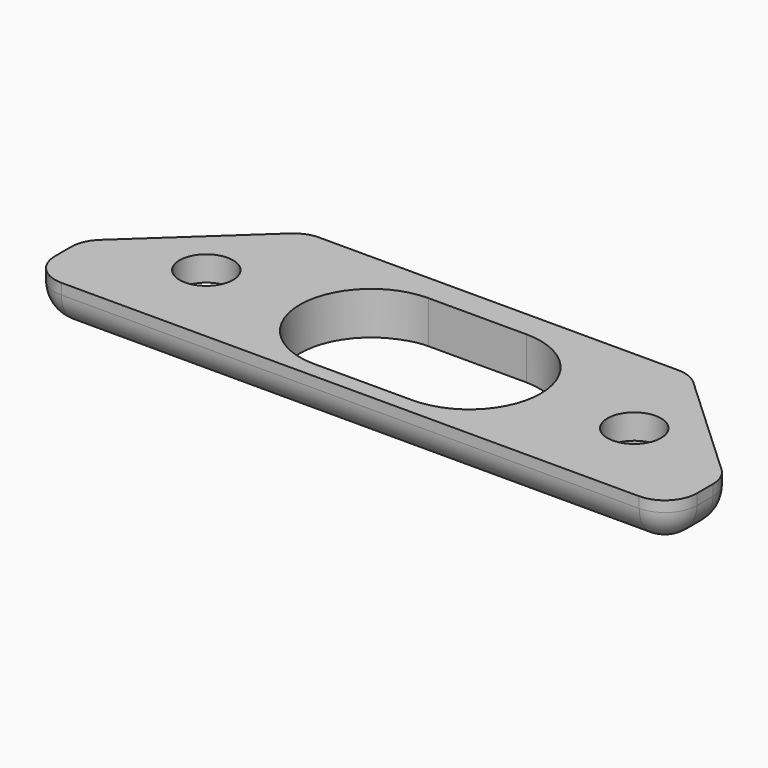
from build123d import *

# Parameters (mm, degrees)
F0_R         = 3
F0_R_2       = 1.5
F1_DEPTH     = 2.4
F2_DEPTH     = 1
F3_T1_DEPTH  = 1.1190522621
F3_T3_DEPTH  = 32.4
F3_T5_DEPTH  = 20.138628613
F3_T7_DEPTH  = 2.365520331
F3_T9_DEPTH  = 8.3614446785
F3_T11_DEPTH = 8.3614446785
F3_T13_DEPTH = 5.1
F3_T15_DEPTH = 2.5639483811
F3_T20_DEPTH = 1.8
F3_S25_W     = 1.8
F3_S25_H     = 1.8
F3_T26_DEPTH = 1.8
F3_S31_W     = 1.8
F3_S31_H     = 1.8
F3_T32_DEPTH = 1.8
F3_T38_DEPTH = 1.8
F3_T44_DEPTH = 1.8
F3_T50_DEPTH = 1.8


# Not quite as in the source:
# - a fillet or chamfer that OpenCascade refuses, or shapes differently, is made with other operations: its cross-section is extruded or revolved along the edge and cut away or added


with BuildPart() as f1:
    # F0 (on Top) → F1 (new body)
    with BuildSketch(Plane.XY):
        Polygon((-18, -1.2002319389), (-18, -4.9048635534), (18, -4.9048635534), (18, -1.2002319389), (10.7755224389, 5.5), (-10.7755224389, 5.5), align=None)
        with Locations((-12, 0)):
            Circle(F0_R, mode=Mode.SUBTRACT)
        with BuildLine():
            ThreePointArc((-2.75, -4), (-6.75, 0), (-2.75, 4))
            Line((-2.75, 4), (2.75, 4))
            ThreePointArc((2.75, 4), (6.75, 0), (2.75, -4))
            Line((2.75, -4), (-2.75, -4))
        make_face(mode=Mode.SUBTRACT)
        with Locations((12, 0)):
            Circle(F0_R, mode=Mode.SUBTRACT)
        with Locations((-12, 0)):
            Circle(F0_R)
        with Locations((-12, 0)):
            Circle(F0_R_2, mode=Mode.SUBTRACT)
        with Locations((12, 0)):
            Circle(F0_R)
        with Locations((12, 0)):
            Circle(F0_R_2, mode=Mode.SUBTRACT)
    extrude(amount=F1_DEPTH)

    # F0 (on Top) → F2 (cut)
    with BuildSketch(Plane.XY):
        with Locations((12, 0)):
            Circle(F0_R)
        with Locations((12, 0)):
            Circle(F0_R_2, mode=Mode.SUBTRACT)
        with Locations((-12, 0)):
            Circle(F0_R)
        with Locations((-12, 0)):
            Circle(F0_R_2, mode=Mode.SUBTRACT)
    extrude(amount=F2_DEPTH, mode=Mode.SUBTRACT)

    # F3: fillet of radius 1.8 on 12 edges, made by hand

    # F3_s2 → F3_t1 (cut)
    with BuildSketch(Plane.XZ.offset(1.9858112913)):
        with BuildLine():
            ThreePointArc((-18, 1.8), (-17.4727922061, 0.5272077939), (-16.2, 0))
            Line((-16.2, 0), (-18, 0))
            Line((-18, 0), (-18, 1.8))
        make_face()
        with BuildLine():
            ThreePointArc((16.2, 0), (17.4727922061, 0.5272077939), (18, 1.8))
            Line((18, 1.8), (18, 0))
            Line((18, 0), (16.2, 0))
        make_face()
    extrude(amount=F3_T1_DEPTH, mode=Mode.SUBTRACT)

    # F3_s4 → F3_t3 (cut)
    with BuildSketch(Plane.YZ.offset(-16.2)):
        with BuildLine():
            ThreePointArc((-4.9048635534, 1.8), (-4.3776557595, 0.5272077939), (-3.1048635534, 0))
            Line((-3.1048635534, 0), (-4.9048635534, 0))
            Line((-4.9048635534, 0), (-4.9048635534, 1.8))
        make_face()
    extrude(amount=F3_T3_DEPTH, mode=Mode.SUBTRACT)

    # F3_s6 → F3_t5 (cut)
    with BuildSketch(Plane.YZ.offset(-10.0693143065)):
        with BuildLine():
            ThreePointArc((3.7, 0), (4.9727922061, 0.5272077939), (5.5, 1.8))
            Line((5.5, 1.8), (5.5, 0))
            Line((5.5, 0), (3.7, 0))
        make_face()
    extrude(amount=F3_T5_DEPTH, mode=Mode.SUBTRACT)

    # F3_s8 → F3_t7 (cut)
    with BuildSketch(Plane.XY.offset(1.8)):
        with BuildLine():
            ThreePointArc((10.0693143065, 5.5), (10.7267347006, 5.3756486581), (11.2933205301, 5.0197760282))
            Line((11.2933205301, 5.0197760282), (10.7755224389, 5.5))
            Line((10.7755224389, 5.5), (10.0693143065, 5.5))
        make_face()
        with BuildLine():
            ThreePointArc((-11.2933205301, 5.0197760282), (-10.7267347006, 5.3756486581), (-10.0693143065, 5.5))
            Line((-10.0693143065, 5.5), (-10.7755224389, 5.5))
            Line((-10.7755224389, 5.5), (-11.2933205301, 5.0197760282))
        make_face()
    extrude(amount=F3_T7_DEPTH, mode=Mode.SUBTRACT)

    # F3_s10 → F3_t9 (cut)
    with BuildSketch(Plane(origin=(-3.5684530391, -3.3095075488, 0), x_dir=(0, 0, 1), z_dir=(-0.7332089046, -0.6800034575, 0))):
        with BuildLine():
            ThreePointArc((1.8, 11.3600414903), (0.5272077939, 10.8328336964), (0, 9.5600414903))
            Line((0, 9.5600414903), (0, 11.3600414903))
            Line((0, 11.3600414903), (1.8, 11.3600414903))
        make_face()
    extrude(amount=F3_T9_DEPTH, mode=Mode.SUBTRACT)

    # F3_s12 → F3_t11 (cut)
    with BuildSketch(Plane(origin=(9.6991387326, -8.9953188401, 0), x_dir=(0, 0, 1), z_dir=(-0.7332089046, 0.6800034575, 0))):
        with BuildLine():
            ThreePointArc((0, 9.5600414903), (0.5272077939, 10.8328336964), (1.8, 11.3600414903))
            Line((1.8, 11.3600414903), (0, 11.3600414903))
            Line((0, 11.3600414903), (0, 9.5600414903))
        make_face()
    extrude(amount=F3_T11_DEPTH, mode=Mode.SUBTRACT)

    # F3_s14 → F3_t13 (cut)
    with BuildSketch(Plane.XY.offset(1.8)):
        with BuildLine():
            ThreePointArc((-18, -3.1048635534), (-17.4727922061, -4.3776557595), (-16.2, -4.9048635534))
            Line((-16.2, -4.9048635534), (-18, -4.9048635534))
            Line((-18, -4.9048635534), (-18, -3.1048635534))
        make_face()
        with BuildLine():
            ThreePointArc((16.2, -4.9048635534), (17.4727922061, -4.3776557595), (18, -3.1048635534))
            Line((18, -3.1048635534), (18, -4.9048635534))
            Line((18, -4.9048635534), (16.2, -4.9048635534))
        make_face()
    extrude(amount=F3_T13_DEPTH, mode=Mode.SUBTRACT)

    # F3_s16 → F3_t15 (cut)
    with BuildSketch(Plane.XY.offset(1.8)):
        with BuildLine():
            ThreePointArc((-18, -1.9858112913), (-17.8497289478, -1.265815181), (-17.4240062235, -0.666035263))
            Line((-17.4240062235, -0.666035263), (-18, -1.2002319389))
            Line((-18, -1.2002319389), (-18, -1.9858112913))
        make_face()
        with BuildLine():
            ThreePointArc((18, -1.9858112913), (17.8497289478, -1.265815181), (17.4240062235, -0.666035263))
            Line((17.4240062235, -0.666035263), (18, -1.2002319389))
            Line((18, -1.2002319389), (18, -1.9858112913))
        make_face()
    extrude(amount=F3_T15_DEPTH, mode=Mode.SUBTRACT)


with BuildPart() as f3_tool18:
    # F3_s19 → F3_t20 (new body)
    with BuildSketch(Plane.XY.offset(1.8)):
        Polygon((-16.2, -1.9858112913), (-18, -1.9858112913), (-18, -1.2002319389), (-17.4240062235, -0.666035263), align=None)
    extrude(amount=-F3_T20_DEPTH)

    # F3_s21 → F3_t22 (revolve, cut)
    with BuildSketch(Plane(origin=(-16.2, -1.9858112913, 1.8), x_dir=(0.9165160821, -0.399997839, 0), z_dir=(0.399997839, 0.9165160821, 0))):
        with BuildLine():
            ThreePointArc((0, -1.8), (1.8, 0), (0, 1.8))
            Line((0, 1.8), (0, -1.8))
        make_face()
    revolve(axis=Axis((-16.2, -1.9858112913, 1.8), (0, 0, -1)), mode=Mode.SUBTRACT)


with BuildPart() as f1_1:
    add(f1.part)

    # F3_t17: cut F3_tool18
    add(f3_tool18.part, mode=Mode.SUBTRACT)


with BuildPart() as f3_tool24:
    # F3_s25 → F3_t26 (new body)
    with BuildSketch(Plane.YZ.offset(-16.2)):
        with Locations((-4.0048635534, 0.9)):
            Rectangle(F3_S25_W, F3_S25_H)
    extrude(amount=-F3_T26_DEPTH)

    # F3_s27 → F3_t28 (revolve, cut)
    with BuildSketch(Plane(origin=(-16.2, -3.1048635534, 1.8), x_dir=(0, 0.7071067812, 0.7071067812), z_dir=(0, -0.7071067812, 0.7071067812))):
        with BuildLine():
            ThreePointArc((0, -1.8), (1.8, 0), (0, 1.8))
            Line((0, 1.8), (0, -1.8))
        make_face()
    revolve(axis=Axis((-16.2, -3.1048635534, 1.8), (-1, 0, 0)), mode=Mode.SUBTRACT)


with BuildPart() as f1_2:
    add(f1_1.part)

    # F3_t23: cut F3_tool24
    add(f3_tool24.part, mode=Mode.SUBTRACT)


with BuildPart() as f3_tool30:
    # F3_s31 → F3_t32 (new body)
    with BuildSketch(Plane.XZ.offset(3.1048635534)):
        with Locations((17.1, 0.9)):
            Rectangle(F3_S31_W, F3_S31_H)
    extrude(amount=F3_T32_DEPTH)

    # F3_s33 → F3_t34 (revolve, cut)
    with BuildSketch(Plane(origin=(16.2, -3.1048635534, 1.8), x_dir=(-0.7071067812, 0, 0.7071067812), z_dir=(0.7071067812, 0, 0.7071067812))):
        with BuildLine():
            ThreePointArc((0, -1.8), (1.8, 0), (0, 1.8))
            Line((0, 1.8), (0, -1.8))
        make_face()
    revolve(axis=Axis((16.2, -3.1048635534, 1.8), (0, -1, 0)), mode=Mode.SUBTRACT)


with BuildPart() as f1_3:
    add(f1_2.part)

    # F3_t29: cut F3_tool30
    add(f3_tool30.part, mode=Mode.SUBTRACT)


with BuildPart() as f3_tool36:
    # F3_s37 → F3_t38 (new body)
    with BuildSketch(Plane.XY.offset(1.8)):
        Polygon((16.2, -1.9858112913), (18, -1.9858112913), (18, -1.2002319389), (17.4240062235, -0.666035263), align=None)
    extrude(amount=-F3_T38_DEPTH)

    # F3_s39 → F3_t40 (revolve, cut)
    with BuildSketch(Plane(origin=(16.2, -1.9858112913, 1.8), x_dir=(-0.9165160821, -0.399997839, 0), z_dir=(0.399997839, -0.9165160821, 0))):
        with BuildLine():
            ThreePointArc((0, -1.8), (1.8, 0), (0, 1.8))
            Line((0, 1.8), (0, -1.8))
        make_face()
    revolve(axis=Axis((16.2, -1.9858112913, 1.8), (0, 0, -1)), mode=Mode.SUBTRACT)


with BuildPart() as f1_4:
    add(f1_3.part)

    # F3_t35: cut F3_tool36
    add(f3_tool36.part, mode=Mode.SUBTRACT)


with BuildPart() as f3_tool42:
    # F3_s43 → F3_t44 (new body)
    with BuildSketch(Plane.XY.offset(1.8)):
        Polygon((10.0693143065, 3.7), (10.0693143065, 5.5), (10.7755224389, 5.5), (11.2933205301, 5.0197760282), align=None)
    extrude(amount=-F3_T44_DEPTH)

    # F3_s45 → F3_t46 (revolve, cut)
    with BuildSketch(Plane(origin=(10.0693143065, 3.7, 1.8), x_dir=(-0.3652335523, -0.9309159212, 0), z_dir=(0.9309159212, -0.3652335523, 0))):
        with BuildLine():
            ThreePointArc((0, -1.8), (1.8, 0), (0, 1.8))
            Line((0, 1.8), (0, -1.8))
        make_face()
    revolve(axis=Axis((10.0693143065, 3.7, 1.8), (0, 0, -1)), mode=Mode.SUBTRACT)


with BuildPart() as f1_5:
    add(f1_4.part)

    # F3_t41: cut F3_tool42
    add(f3_tool42.part, mode=Mode.SUBTRACT)


with BuildPart() as f3_tool48:
    # F3_s49 → F3_t50 (new body)
    with BuildSketch(Plane.XY.offset(1.8)):
        Polygon((-10.0693143065, 3.7), (-10.0693143065, 5.5), (-10.7755224389, 5.5), (-11.2933205301, 5.0197760282), align=None)
    extrude(amount=-F3_T50_DEPTH)

    # F3_s51 → F3_t52 (revolve, cut)
    with BuildSketch(Plane(origin=(-10.0693143065, 3.7, 1.8), x_dir=(0.3652335523, -0.9309159212, 0), z_dir=(0.9309159212, 0.3652335523, 0))):
        with BuildLine():
            ThreePointArc((0, -1.8), (1.8, 0), (0, 1.8))
            Line((0, 1.8), (0, -1.8))
        make_face()
    revolve(axis=Axis((-10.0693143065, 3.7, 1.8), (0, 0, -1)), mode=Mode.SUBTRACT)


with BuildPart() as f1_6:
    add(f1_5.part)

    # F3_t47: cut F3_tool48
    add(f3_tool48.part, mode=Mode.SUBTRACT)


solid = f1_6.part
